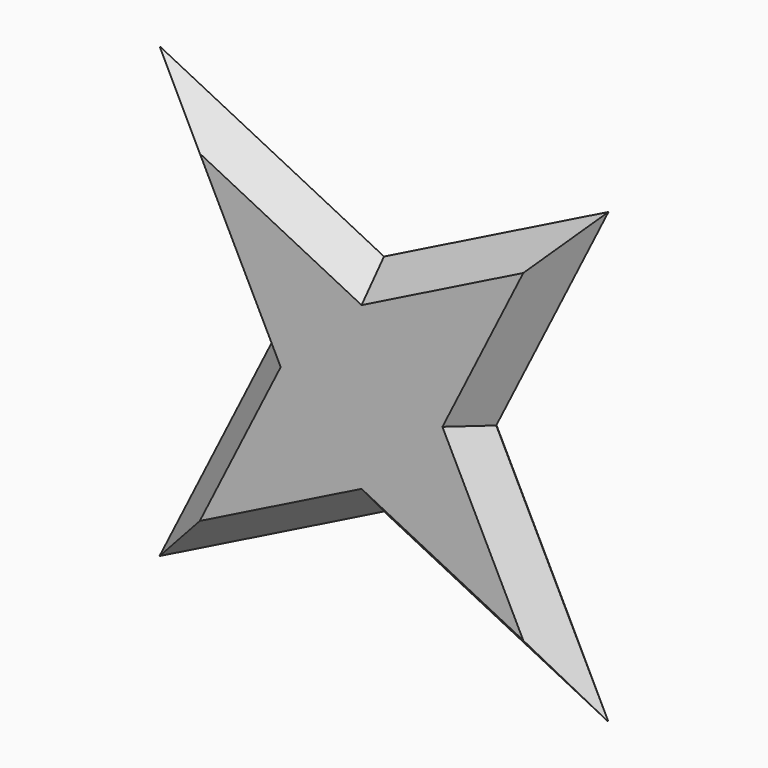
from build123d import *

# Parameters (mm, degrees)
F1_DEPTH = 6.35
F2_SIZE  = 3.175
F3_SIZE  = 3.17499


# Not quite as in the source:
# - a fillet or chamfer is up to 0.001 mm smaller than in the source, because OpenCascade refuses the exact size


with BuildPart() as f1:
    # F0 (on Front) → F1 (new body)
    with BuildSketch(Plane.XZ):
        Polygon((0, 12.7), (-25.4, 25.4), (-12.7, 0), (-25.4, -25.4), (0, -12.7), (25.4, -25.4), (12.7, 0), (25.4, 25.4), align=None)
    extrude(amount=F1_DEPTH)

    # F2
    f2_edges = [f1.edges().sort_by_distance(p)[0] for p in [
        (-19.05, -6.35, 12.7),
        (-12.7, -6.35, 19.05),
        (12.7, -6.35, -19.05),
        (19.05, -6.35, -12.7),
        (19.05, -6.35, 12.7),
        (12.7, -6.35, 19.05),
        (-19.05, -6.35, -12.7),
        (-12.7, -6.35, -19.05),
    ]]
    chamfer(f2_edges, length=F2_SIZE)

    # F3 (size 3.175 in the source; OpenCascade refuses exactly that, so slightly less here)
    f3_edges = [f1.edges().sort_by_distance(p)[0] for p in [
        (-19.05, 0, -12.7),
        (-12.7, 0, -19.05),
        (12.7, 0, -19.05),
        (19.05, 0, -12.7),
        (19.05, 0, 12.7),
        (12.7, 0, 19.05),
        (-12.7, 0, 19.05),
        (-19.05, 0, 12.7),
    ]]
    chamfer(f3_edges, length=F3_SIZE)


solid = f1.part
